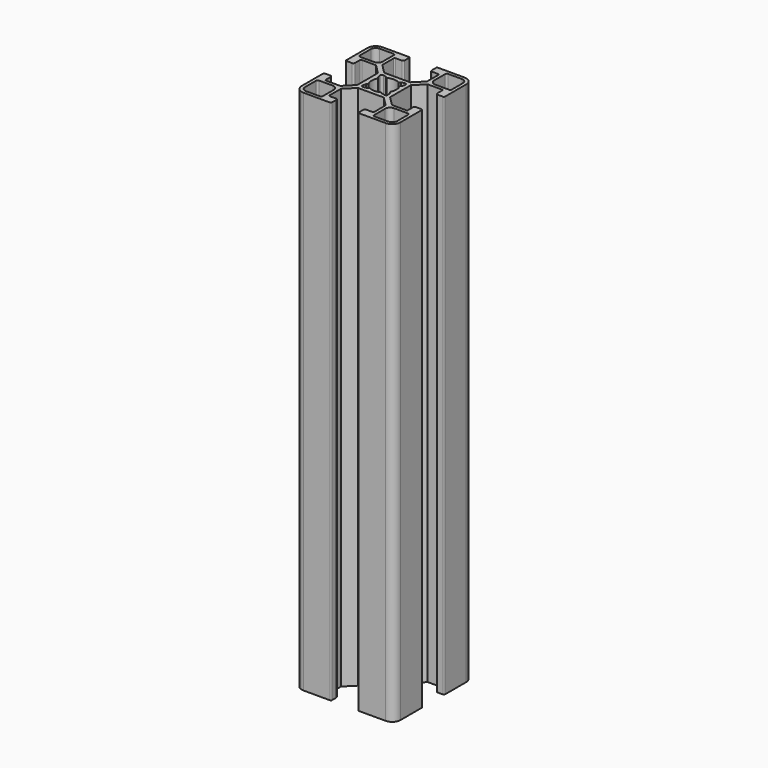
from build123d import *

# Parameters (mm, degrees)
F1_DEPTH = 160


# Not quite as in the source:
# - ends of sketch curves that miss each other by under 0.0002 mm in the source are joined
# - the program builds the solid bodies; features that only make, move or delete a surface that nothing else refers to are left out


with BuildPart() as f1:
    # F0 (on Top) → F1 (new body)
    with BuildSketch(Plane.XY):
        with BuildLine():
            Line((3.939341, -5), (6.799995, -7.860656))
            Line((6.799995, -7.860656), (6.799995, -12.199997))
            ThreePointArc((6.799995, -12.199997), (6.7121307415, -12.4121300846), (6.5, -12.5))
            Line((6.5, -12.5), (4.599998, -12.5))
            ThreePointArc((4.599998, -12.5), (4.2464446094, -12.6464466094), (4.099998, -13))
            Line((4.099998, -13), (4.099998, -14.699997))
            ThreePointArc((4.099998, -14.699997), (4.1878632585, -14.9121300846), (4.399994, -15))
            Line((4.399994, -15), (12.5, -15))
            ThreePointArc((12.5, -15), (14.267766953, -14.267766953), (15, -12.5))
            Line((15, -12.5), (15, -4.399994))
            ThreePointArc((15, -4.399994), (14.9121300846, -4.1878632585), (14.699997, -4.099999))
            Line((14.699997, -4.099999), (13, -4.099998))
            ThreePointArc((13, -4.099998), (12.6464466094, -4.2464446094), (12.5, -4.599998))
            Line((12.5, -4.599998), (12.5, -6.5))
            ThreePointArc((12.5, -6.5), (12.4121300846, -6.7121307415), (12.199997, -6.799995))
            Line((12.199997, -6.799995), (7.860655, -6.799995))
            Line((7.860655, -6.799995), (5, -3.93934))
            Line((5, -3.93934), (5, 3.939341))
            Line((5, 3.939341), (7.860655, 6.799995))
            Line((7.860655, 6.799995), (12.199997, 6.799995))
            ThreePointArc((12.199997, 6.799995), (12.4121300846, 6.7121307415), (12.5, 6.5))
            Line((12.5, 6.5), (12.5, 4.599998))
            ThreePointArc((12.5, 4.599998), (12.6464466094, 4.2464446094), (13, 4.099998))
            Line((13, 4.099998), (14.699997, 4.099998))
            ThreePointArc((14.699997, 4.099998), (14.9121300846, 4.1878632585), (15, 4.399994))
            Line((15, 4.399994), (15, 12.5))
            ThreePointArc((15, 12.5), (14.267766953, 14.267766953), (12.5, 15))
            Line((12.5, 15), (4.399994, 15))
            ThreePointArc((4.399994, 15), (4.1878632585, 14.9121300846), (4.099999, 14.699997))
            Line((4.099999, 14.699997), (4.099998, 13))
            ThreePointArc((4.099998, 13), (4.2464446094, 12.6464466094), (4.599998, 12.5))
            Line((4.599998, 12.5), (6.5, 12.5))
            ThreePointArc((6.5, 12.5), (6.7121307415, 12.4121300846), (6.799995, 12.199997))
            Line((6.799995, 12.199997), (6.799995, 7.860655))
            Line((6.799995, 7.860655), (3.939341, 5))
            Line((3.939341, 5), (-3.93934, 5))
            Line((-3.93934, 5), (-6.799995, 7.860655))
            Line((-6.799995, 7.860655), (-6.799995, 12.199997))
            ThreePointArc((-6.799995, 12.199997), (-6.7121307415, 12.4121300846), (-6.5, 12.5))
            Line((-6.5, 12.5), (-4.599998, 12.5))
            ThreePointArc((-4.599998, 12.5), (-4.2464446094, 12.6464466094), (-4.099998, 13))
            Line((-4.099998, 13), (-4.099998, 14.699997))
            ThreePointArc((-4.099998, 14.699997), (-4.1878632585, 14.9121300846), (-4.399994, 15))
            Line((-4.399994, 15), (-12.5, 15))
            ThreePointArc((-12.5, 15), (-14.267766953, 14.267766953), (-15, 12.5))
            Line((-15, 12.5), (-15, 4.399994))
            ThreePointArc((-15, 4.399994), (-14.9121300846, 4.1878632585), (-14.699997, 4.099999))
            Line((-14.699997, 4.099999), (-13, 4.099998))
            ThreePointArc((-13, 4.099998), (-12.6464466094, 4.2464446094), (-12.5, 4.599998))
            Line((-12.5, 4.599998), (-12.5, 6.5))
            ThreePointArc((-12.5, 6.5), (-12.4121300846, 6.7121307415), (-12.199997, 6.799995))
            Line((-12.199997, 6.799995), (-7.860656, 6.799995))
            Line((-7.860656, 6.799995), (-5, 3.939341))
            Line((-5, 3.939341), (-5, -3.93934))
            Line((-5, -3.93934), (-7.860656, -6.799995))
            Line((-7.860656, -6.799995), (-12.199997, -6.799995))
            ThreePointArc((-12.199997, -6.799995), (-12.4121300846, -6.7121307415), (-12.5, -6.5))
            Line((-12.5, -6.5), (-12.5, -4.599998))
            ThreePointArc((-12.5, -4.599998), (-12.6464466094, -4.2464446094), (-13, -4.099998))
            Line((-13, -4.099998), (-14.699997, -4.099998))
            ThreePointArc((-14.699997, -4.099998), (-14.9121300846, -4.1878632585), (-15, -4.399994))
            Line((-15, -4.399994), (-15, -12.5))
            ThreePointArc((-15, -12.5), (-14.267766953, -14.267766953), (-12.5, -15))
            Line((-12.5, -15), (-4.399994, -15))
            ThreePointArc((-4.399994, -15), (-4.1878632585, -14.9121300846), (-4.099999, -14.699997))
            Line((-4.099999, -14.699997), (-4.099998, -13))
            ThreePointArc((-4.099998, -13), (-4.2464446094, -12.6464466094), (-4.599998, -12.5))
            Line((-4.599998, -12.5), (-6.5, -12.5))
            ThreePointArc((-6.5, -12.5), (-6.7121307415, -12.4121300846), (-6.799995, -12.199997))
            Line((-6.799995, -12.199997), (-6.799995, -7.860656))
            Line((-6.799995, -7.860656), (-3.93934, -5))
            Line((-3.93934, -5), (3.939341, -5))
        make_face()
        with BuildLine():
            Line((-8.299995, -14), (-12.5, -14))
            ThreePointArc((-12.5, -14), (-13.5606601718, -13.5606601718), (-14, -12.5))
            Line((-14, -12.5), (-14, -8.299995))
            ThreePointArc((-14, -8.299995), (-13.8535533906, -7.9464416094), (-13.5, -7.799995))
            Line((-13.5, -7.799995), (-9.299995, -7.799995))
            ThreePointArc((-9.299995, -7.799995), (-8.2393348282, -8.2393348282), (-7.799995, -9.299995))
            Line((-7.799995, -9.299995), (-7.799995, -13.5))
            ThreePointArc((-7.799995, -13.5), (-7.9464416094, -13.8535533906), (-8.299995, -14))
        make_face(mode=Mode.SUBTRACT)
        with BuildLine():
            Line((12.5, -14), (8.299995, -14))
            ThreePointArc((8.299995, -14), (7.9464416094, -13.8535533906), (7.799995, -13.5))
            Line((7.799995, -13.5), (7.799995, -9.299995))
            ThreePointArc((7.799995, -9.299995), (8.2393348282, -8.2393348282), (9.299995, -7.799995))
            Line((9.299995, -7.799995), (13.5, -7.799995))
            ThreePointArc((13.5, -7.799995), (13.8535533906, -7.9464416094), (14, -8.299995))
            Line((14, -8.299995), (14, -12.5))
            ThreePointArc((14, -12.5), (13.5606601718, -13.5606601718), (12.5, -14))
        make_face(mode=Mode.SUBTRACT)
        with BuildLine():
            Line((3.657288, -2.243073), (3.878887, -3.285876))
            ThreePointArc((3.878887, -3.285876), (3.7433613906, -3.7433613906), (3.2858769836, -3.8788870773))
            Line((3.2858769836, -3.8788870773), (2.243074, -3.657287))
            Line((2.243074, -3.657287), (2.005135, -3.419348))
            ThreePointArc((2.005135, -3.419348), (1.841799908, -3.3354753308), (1.6601868142, -3.3624816237))
            ThreePointArc((1.6601868142, -3.3624816237), (0, -3.75), (-1.6601870383, -3.3624810777))
            ThreePointArc((-1.6601870383, -3.3624810777), (-1.841799908, -3.3354753308), (-2.0051340344, -3.4193479656))
            Line((-2.0051340344, -3.4193479656), (-2.243073, -3.657287))
            Line((-2.243073, -3.657287), (-3.285876, -3.878887))
            ThreePointArc((-3.285876, -3.878887), (-3.7433613906, -3.7433613906), (-3.8788870773, -3.2858769836))
            Line((-3.8788870773, -3.2858769836), (-3.657287, -2.243073))
            Line((-3.657287, -2.243073), (-3.419348, -2.005134))
            ThreePointArc((-3.419348, -2.005134), (-3.3354753308, -1.841799908), (-3.3624816237, -1.6601868142))
            ThreePointArc((-3.3624816237, -1.6601868142), (-3.75, 0), (-3.3624810777, 1.6601870383))
            ThreePointArc((-3.3624810777, 1.6601870383), (-3.3354753883, 1.8418002569), (-3.4193484656, 2.0051345344))
            Line((-3.4193484656, 2.0051345344), (-3.657287, 2.243074))
            Line((-3.657287, 2.243074), (-3.878887, 3.285877))
            ThreePointArc((-3.878887, 3.285877), (-3.7433613906, 3.7433613906), (-3.2858769836, 3.8788870773))
            Line((-3.2858769836, 3.8788870773), (-2.243073, 3.657288))
            Line((-2.243073, 3.657288), (-2.005134, 3.419348))
            ThreePointArc((-2.005134, 3.419348), (-1.8418001264, 3.3354753668), (-1.6601872112, 3.3624814277))
            ThreePointArc((-1.6601872112, 3.3624814277), (0, 3.75), (1.6601870383, 3.3624810777))
            ThreePointArc((1.6601870383, 3.3624810777), (1.8418002569, 3.3354753883), (2.0051345344, 3.4193484656))
            Line((2.0051345344, 3.4193484656), (2.243074, 3.657288))
            Line((2.243074, 3.657288), (3.285877, 3.878887))
            ThreePointArc((3.285877, 3.878887), (3.7433610448, 3.7433617364), (3.8788872806, 3.2858779404))
            Line((3.8788872806, 3.2858779404), (3.657288, 2.243074))
            Line((3.657288, 2.243074), (3.419348, 2.005135))
            ThreePointArc((3.419348, 2.005135), (3.3354753668, 1.8418001264), (3.3624814277, 1.6601872112))
            ThreePointArc((3.3624814277, 1.6601872112), (3.75, 0), (3.3624810777, -1.6601870383))
            ThreePointArc((3.3624810777, -1.6601870383), (3.3354753308, -1.841799908), (3.4193479656, -2.0051340344))
            Line((3.4193479656, -2.0051340344), (3.657288, -2.243073))
        make_face(mode=Mode.SUBTRACT)
        with BuildLine():
            Line((-9.299995, 7.799995), (-13.5, 7.799995))
            ThreePointArc((-13.5, 7.799995), (-13.8535533906, 7.9464416094), (-14, 8.299995))
            Line((-14, 8.299995), (-14, 12.5))
            ThreePointArc((-14, 12.5), (-13.5606601718, 13.5606601718), (-12.5, 14))
            Line((-12.5, 14), (-8.299995, 14))
            ThreePointArc((-8.299995, 14), (-7.9464416094, 13.8535533906), (-7.799995, 13.5))
            Line((-7.799995, 13.5), (-7.799995, 9.299995))
            ThreePointArc((-7.799995, 9.299995), (-8.2393348282, 8.2393348282), (-9.299995, 7.799995))
        make_face(mode=Mode.SUBTRACT)
        with BuildLine():
            Line((13.5, 7.799995), (9.299995, 7.799995))
            ThreePointArc((9.299995, 7.799995), (8.2393348282, 8.2393348282), (7.799995, 9.299995))
            Line((7.799995, 9.299995), (7.799995, 13.5))
            ThreePointArc((7.799995, 13.5), (7.9464416094, 13.8535533906), (8.299995, 14))
            Line((8.299995, 14), (12.5, 14))
            ThreePointArc((12.5, 14), (13.5606601718, 13.5606601718), (14, 12.5))
            Line((14, 12.5), (14, 8.299995))
            ThreePointArc((14, 8.299995), (13.8535533906, 7.9464416094), (13.5, 7.799995))
        make_face(mode=Mode.SUBTRACT)
    extrude(amount=F1_DEPTH)


solid = f1.part
